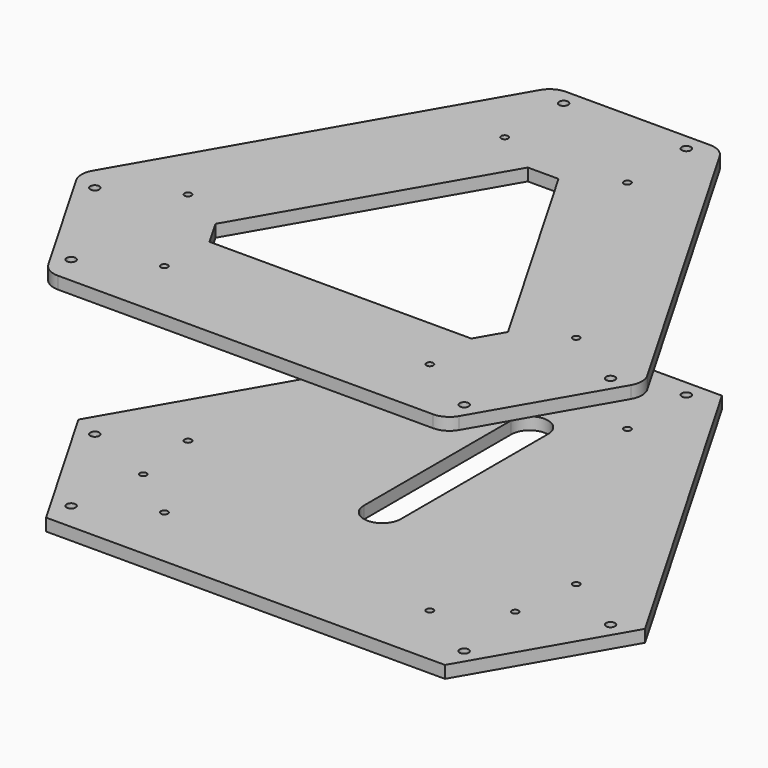
from build123d import *

# Parameters (mm, degrees)
F0_R     = 2.2
F0_R_2   = 1.7
F1_DEPTH = 6
F3_R     = 2.2
F3_R_2   = 1.7
F3_R_3   = 1.65
F4_DEPTH = 6
F5_R     = 10


# Not quite as in the source:
# - a feature names something its author has since deleted; it is built from what else it names


with BuildPart() as f1:
    # F0 (on Top) → F1 (new body)
    with BuildSketch(Plane.XY):
        Polygon((-41, 136.2546635288), (-138.5, -32.6202902092), (-97.5, -103.6343733195), (97.5, -103.6343733195), (138.5, -32.6202902092), (41, 136.2546635288), align=None)
        with Locations((-96.0717967697, -90.1080938779)):
            Circle(F0_R, mode=Mode.SUBTRACT)
        with Locations((-64.8948822335, -72.1080938779)):
            Circle(F0_R_2, mode=Mode.SUBTRACT)
        with Locations((-126.0717967697, -38.1465696508)):
            Circle(F0_R, mode=Mode.SUBTRACT)
        with Locations((-94.8948822335, -20.1465696508)):
            Circle(F0_R_2, mode=Mode.SUBTRACT)
        with Locations((64.8948822335, -72.1080938779)):
            Circle(F0_R_2, mode=Mode.SUBTRACT)
        with Locations((96.0717967697, -90.1080938779)):
            Circle(F0_R, mode=Mode.SUBTRACT)
        with Locations((94.8948822335, -20.1465696508)):
            Circle(F0_R_2, mode=Mode.SUBTRACT)
        with Locations((126.0717967697, -38.1465696508)):
            Circle(F0_R, mode=Mode.SUBTRACT)
        with Locations((-30, 92.2546635288)):
            Circle(F0_R_2, mode=Mode.SUBTRACT)
        with Locations((-30, 128.2546635288)):
            Circle(F0_R, mode=Mode.SUBTRACT)
        Polygon((71.527368774, -32.6202902092), (64.013684387, -45.6343733195), (-64.013684387, -45.6343733195), (-71.527368774, -32.6202902092), (-7.513684387, 78.2546635288), (7.513684387, 78.2546635288), align=None, mode=Mode.SUBTRACT)
        with Locations((30, 92.2546635288)):
            Circle(F0_R_2, mode=Mode.SUBTRACT)
        with Locations((30, 128.2546635288)):
            Circle(F0_R, mode=Mode.SUBTRACT)
    extrude(amount=F1_DEPTH)

    # F5
    f5_edges = [f1.edges().sort_by_distance(p)[0] for p in [
        (97.5, -103.634373, 3),
        (138.5, -32.62029, 3),
        (-97.5, -103.634373, 3),
        (-138.5, -32.62029, 3),
        (-41, 136.254664, 3),
        (41, 136.254664, 3),
    ]]
    fillet(f5_edges, radius=F5_R)


with BuildPart() as f4:
    # F3 (on offset) → F4 (new body)
    with BuildSketch(Plane(origin=(0, 0, -100), x_dir=(1, 0, 0), z_dir=(0, 0, -1))):
        Polygon((97.5, 103.6343733195), (-97.5, 103.6343733195), (-138.5, 32.6202902092), (-41, -136.2546635288), (41, -136.2546635288), (138.5, 32.6202902092), align=None)
        with Locations((-30, -128.2546635288)):
            Circle(F3_R, mode=Mode.SUBTRACT)
        with Locations((-30, -92.2546635288)):
            Circle(F3_R_2, mode=Mode.SUBTRACT)
        with Locations((30, -128.2546635288)):
            Circle(F3_R, mode=Mode.SUBTRACT)
        with Locations((0, -105)):
            Circle(F3_R_3, mode=Mode.SUBTRACT)
        with Locations((30, -92.2546635288)):
            Circle(F3_R_2, mode=Mode.SUBTRACT)
        with BuildLine():
            Line((-9, -70), (-9, 20))
            ThreePointArc((-9, 20), (0, 29), (9, 20))
            Line((9, 20), (9, -70))
            ThreePointArc((9, -70), (0, -79), (-9, -70))
        make_face(mode=Mode.SUBTRACT)
        with Locations((-126.0717967697, 38.1465696508)):
            Circle(F3_R, mode=Mode.SUBTRACT)
        with Locations((-94.8948822335, 20.1465696508)):
            Circle(F3_R_2, mode=Mode.SUBTRACT)
        with Locations((-90.9326673974, 52.5)):
            Circle(F3_R_3, mode=Mode.SUBTRACT)
        with Locations((-96.0717967697, 90.1080938779)):
            Circle(F3_R, mode=Mode.SUBTRACT)
        with Locations((-64.8948822335, 72.1080938779)):
            Circle(F3_R_2, mode=Mode.SUBTRACT)
        with Locations((94.8948822335, 20.1465696508)):
            Circle(F3_R_2, mode=Mode.SUBTRACT)
        with Locations((126.0717967697, 38.1465696508)):
            Circle(F3_R, mode=Mode.SUBTRACT)
        with Locations((64.8948822335, 72.1080938779)):
            Circle(F3_R_2, mode=Mode.SUBTRACT)
        with Locations((90.9326673974, 52.5)):
            Circle(F3_R_3, mode=Mode.SUBTRACT)
        with Locations((96.0717967697, 90.1080938779)):
            Circle(F3_R, mode=Mode.SUBTRACT)
    extrude(amount=F4_DEPTH)


solid = Compound([f1.part, f4.part])
